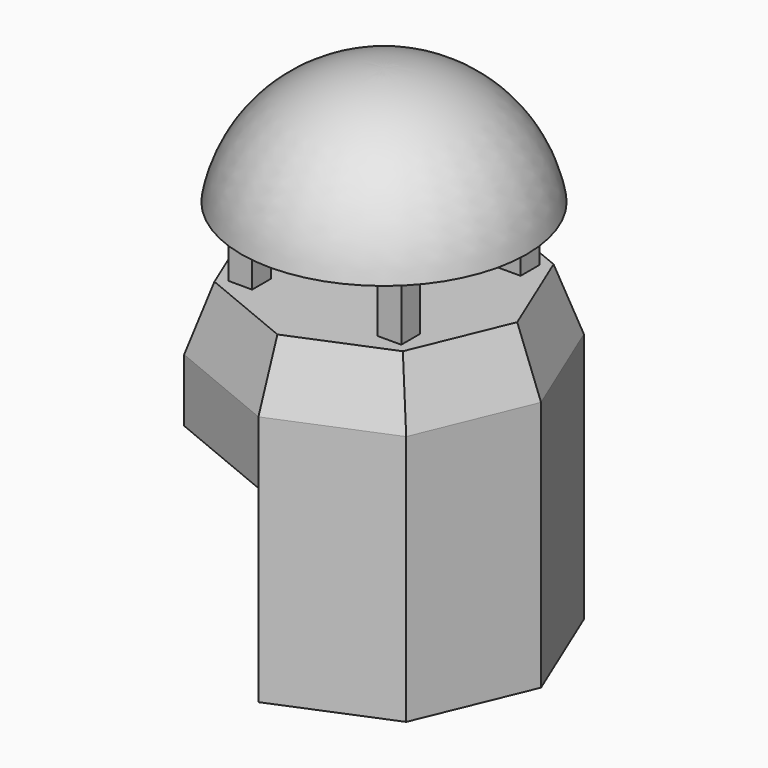
from build123d import *

# Parameters (mm, degrees)
F2_DEPTH  = 60.96
F4_DEPTH  = 20.32
F9_W      = 7.62
F9_H      = 7.62
F14_DEPTH = 20.32


with BuildPart() as f2:
    # F0 (on Top) → F2 (new body)
    with BuildSketch(Plane.XY):
        Polygon((35.9210244843, 35.9210244843), (0, 50.8), (0, -50.8), (35.9210244843, -35.9210244843), (50.8, 0), align=None)
    extrude(amount=F2_DEPTH)

    # F3 (on offset) → F4 (join)
    with BuildSketch(Plane.XY.offset(60.96)):
        Polygon((35.9210244843, 35.9210244843), (0, 50.8), (-35.9210244843, 35.9210244843), (-50.8, 0), (-35.9210244843, -35.9210244843), (0, -50.8), (35.9210244843, -35.9210244843), (50.8, 0), align=None)
    extrude(amount=F4_DEPTH)

    # F7 (on offset) → F13 section 0
    with BuildSketch(Plane.XY.offset(81.28)):
        Polygon((0, 50.8), (-35.9210244843, 35.9210244843), (-50.8, 0), (-35.9210244843, -35.9210244843), (0, -50.8), (35.9210244843, -35.9210244843), (50.8, 0), (35.9210244843, 35.9210244843), align=None)
    # F8 (on offset) → F13 section 1
    with BuildSketch(Plane.XY.offset(101.6)):
        Polygon((43.1052293811, 0), (30.48, 30.48), (0, 43.1052293811), (-30.48, 30.48), (-43.1052293811, 0), (-30.48, -30.48), (0, -43.1052293811), (30.48, -30.48), align=None)
    loft()

    # F9 (on offset) → F14 (join)
    with BuildSketch(Plane.XY.offset(101.6)):
        with Locations((-24.13, 24.13)):
            Rectangle(F9_W, F9_H)
        with Locations((24.13, 24.13)):
            Rectangle(F9_W, F9_H)
        with Locations((-24.13, -24.13)):
            Rectangle(F9_W, F9_H)
        with Locations((24.13, -24.13)):
            Rectangle(F9_W, F9_H)
    extrude(amount=F14_DEPTH)

    # F15 (on Front) → F16 (revolve)
    with BuildSketch(Plane.XZ):
        with BuildLine():
            ThreePointArc((0, 160.02), (-30.0961069105, 149.4685742909), (-46.1642209939, 121.92))
            Line((-46.1642209939, 121.92), (0, 121.92))
            Line((0, 121.92), (0, 160.02))
        make_face()
    revolve(axis=Axis((0, 0, 140.97), (0, 0, 1)))


solid = f2.part
